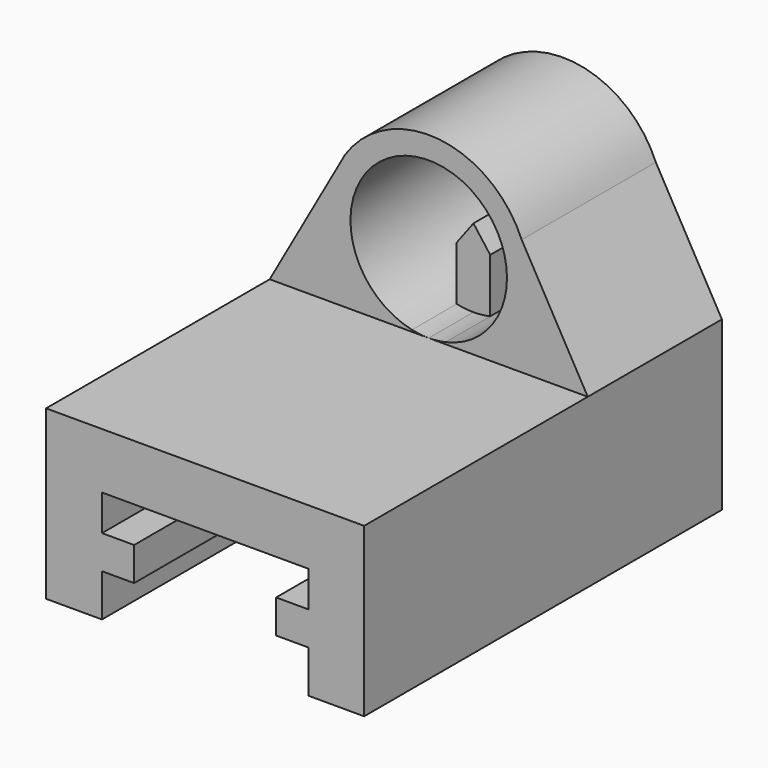
from build123d import *
from build123d import SkipClean  # not in build123d's __all__

# Parameters (mm, degrees)
F0_W     = 2.875
F0_H     = 3
F1_DEPTH = 40
F2_DEPTH = 15
F3_DEPTH = 10
F4_DEPTH = 15
F5_DEPTH = 5


with BuildPart() as f1:
    # F0 (on Front) → F1 (new body)
    with BuildSketch(Plane.XZ):
        Polygon((-9.225, 4.615817529), (-9.225, 8.415817529), (-9.225, 11.415817529), (-9.225, 14.615817529), (9.225, 14.615817529), (9.225, 11.415817529), (9.225, 8.415817529), (9.225, 4.615817529), (14.225, 4.615817529), (14.225, 19.615817529), (5.6568542495, 19.615817529), (1.5, 19.615817529), (0, 19.615817529), (-1.5, 19.615817529), (-5.6568542495, 19.615817529), (-14.225, 19.615817529), (-14.225, 4.615817529), align=None)
        with Locations((-7.7875, 9.915817529)):
            Rectangle(F0_W, F0_H)
        with Locations((7.7875, 9.915817529)):
            Rectangle(F0_W, F0_H)
    extrude(amount=F1_DEPTH)

    # F0 (on Front) → F2 (join)
    with BuildSketch(Plane.XZ):
        with BuildLine():
            Line((-8.1629870472, 30.4060210151), (-14.225, 19.615817529))
            Line((-14.225, 19.615817529), (-5.6568542495, 19.615817529))
            ThreePointArc((-5.6568542495, 19.615817529), (-8.766648515, 24.5796756343), (-8.1629870472, 30.4060210151))
        make_face()
        with BuildLine():
            ThreePointArc((-8.1629870472, 30.4060210151), (-8.766648515, 24.5796756343), (-5.6568542495, 19.615817529))
            Line((-5.6568542495, 19.615817529), (-1.5, 19.615817529))
            Line((-1.5, 19.615817529), (-1.5, 19.7784203634))
            ThreePointArc((-1.5, 19.7784203634), (-4.3874821937, 32.0701735863), (7, 26.615817529))
            ThreePointArc((7, 26.615817529), (5.4543560573, 22.2283353353), (1.5, 19.7784203634))
            Line((1.5, 19.7784203634), (1.5, 19.615817529))
            Line((1.5, 19.615817529), (5.6568542495, 19.615817529))
            ThreePointArc((5.6568542495, 19.615817529), (8.7219157357, 24.3958657503), (8.3150665238, 30.0596045005))
            ThreePointArc((8.3150665238, 30.0596045005), (0.8822712117, 35.5724685498), (-7.4833147735, 31.615817529))
            Line((-7.4833147735, 31.615817529), (-8.1629870472, 30.4060210151))
        make_face()
        with BuildLine():
            Line((5.6568542495, 19.615817529), (14.225, 19.615817529))
            Line((14.225, 19.615817529), (8.3150665238, 30.0596045005))
            ThreePointArc((8.3150665238, 30.0596045005), (8.7219157357, 24.3958657503), (5.6568542495, 19.615817529))
        make_face()
    extrude(amount=F2_DEPTH)

    # F0 (on Front) → F3 (join)
    with BuildSketch(Plane.XZ):
        with BuildLine():
            ThreePointArc((-1.5, 19.7784203634), (-0.7543937436, 19.6565869623), (0, 19.615817529))
            ThreePointArc((0, 19.615817529), (0.7543937436, 19.6565869623), (1.5, 19.7784203634))
            Line((1.5, 19.7784203634), (1.5, 24.615817529))
            Line((1.5, 24.615817529), (0, 26.615817529))
            Line((0, 26.615817529), (-1.5, 24.615817529))
            Line((-1.5, 24.615817529), (-1.5, 19.7784203634))
        make_face()
        with BuildLine():
            Line((-1.5, 19.7784203634), (-1.5, 19.615817529))
            Line((-1.5, 19.615817529), (0, 19.615817529))
            ThreePointArc((0, 19.615817529), (-0.7543937436, 19.6565869623), (-1.5, 19.7784203634))
        make_face()
        with BuildLine():
            Line((0, 19.615817529), (1.5, 19.615817529))
            Line((1.5, 19.615817529), (1.5, 19.7784203634))
            ThreePointArc((1.5, 19.7784203634), (0.7543937436, 19.6565869623), (0, 19.615817529))
        make_face()
    extrude(amount=F3_DEPTH)

    # F0 (on Front) → F4 (join)
    with BuildSketch(Plane.XZ):
        with BuildLine():
            Line((0, 19.615817529), (1.5, 19.615817529))
            Line((1.5, 19.615817529), (1.5, 19.7784203634))
            ThreePointArc((1.5, 19.7784203634), (0.7543937436, 19.6565869623), (0, 19.615817529))
        make_face()
        with BuildLine():
            Line((-1.5, 19.7784203634), (-1.5, 19.615817529))
            Line((-1.5, 19.615817529), (0, 19.615817529))
            ThreePointArc((0, 19.615817529), (-0.7543937436, 19.6565869623), (-1.5, 19.7784203634))
        make_face()
    extrude(amount=F4_DEPTH)

    # F0 (on Front) → F5 (cut)
    with BuildSketch(Plane.XZ):
        with BuildLine():
            ThreePointArc((-1.5, 19.7784203634), (-0.7543937436, 19.6565869623), (0, 19.615817529))
            ThreePointArc((0, 19.615817529), (0.7543937436, 19.6565869623), (1.5, 19.7784203634))
            Line((1.5, 19.7784203634), (1.5, 24.615817529))
            Line((1.5, 24.615817529), (0, 26.615817529))
            Line((0, 26.615817529), (-1.5, 24.615817529))
            Line((-1.5, 24.615817529), (-1.5, 19.7784203634))
        make_face()
    with SkipClean():  # cleaning this boolean's faces spoils the solid; the shape is the same uncleaned
        extrude(amount=F5_DEPTH, mode=Mode.SUBTRACT)


solid = f1.part
